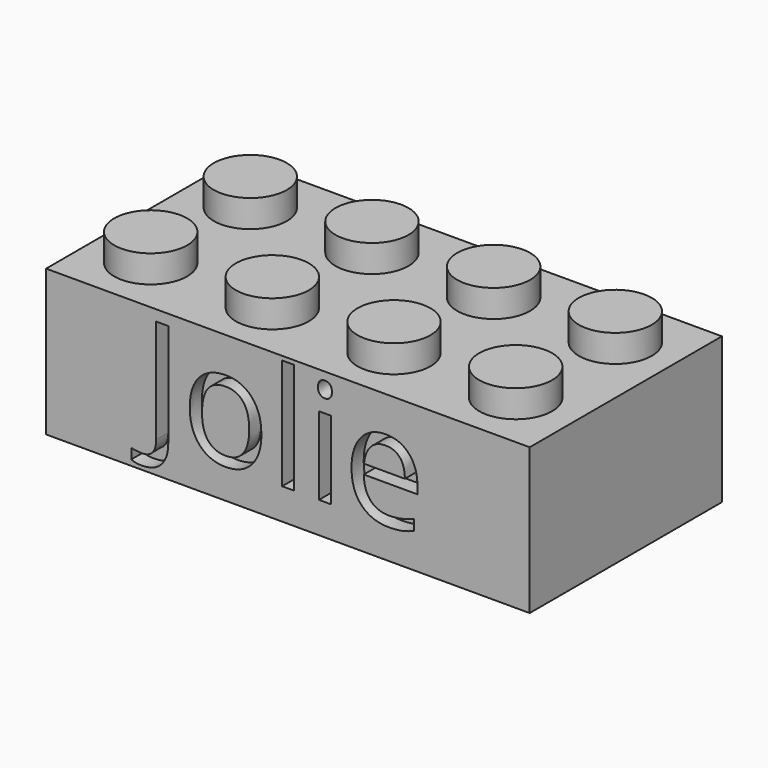
from build123d import *

# Parameters (mm, degrees)
F0_W          = 31.8
F0_H          = 15.8
F1_DEPTH      = 9.6
F2_W          = 29.4
F2_H          = 13.4
F3_DEPTH      = 8.4
F4_R          = 2.4
F5_DEPTH      = 1.8
F7_R          = 1.3
F8_DEPTH      = 1.2
F9_R          = 3.255
F9_R_2        = 2.4
F10_DEPTH     = 8.4
F11_W         = 0.6
F11_H         = 0.3
F12_DEPTH     = 9.6
F15_TEXT_SIZE = 9.5833333333
F16_DEPTH     = 1


# Not quite as in the source:
# - the program builds the solid bodies; features that only make, move or delete a surface that nothing else refers to are left out
# - Text() gives the source's letters only with a copy of the font that has no kerning and outlines rounded to 1/6400 em; it was checked with that copy


with BuildPart() as f1:
    # F0 (on Top) → F1 (new body)
    with BuildSketch(Plane.XY):
        Rectangle(F0_W, F0_H)
    extrude(amount=F1_DEPTH)

    # F2 (on Top) → F3 (cut)
    with BuildSketch(Plane.XY):
        Rectangle(F2_W, F2_H)
    extrude(amount=F3_DEPTH, mode=Mode.SUBTRACT)

    # F4 (on face) → F5 (join)
    with BuildSketch(Plane.XY.offset(9.6)):
        with Locations((-11.95, 3.95)):
            Circle(F4_R)
        with Locations((-12.1022495041, -4.0485511243)):
            Circle(F4_R)
        with Locations((-3.95, 3.95)):
            Circle(F4_R)
        with Locations((-4.1022495041, -4.0485511243)):
            Circle(F4_R)
        with Locations((4.05, 3.95)):
            Circle(F4_R)
        with Locations((3.8977504959, -4.0485511243)):
            Circle(F4_R)
        with Locations((12.05, 3.95)):
            Circle(F4_R)
        with Locations((11.8977504959, -4.0485511243)):
            Circle(F4_R)
    extrude(amount=F5_DEPTH)

    # F7 (on offset) → F8 (cut)
    with BuildSketch(Plane.XY.offset(8.4)):
        with Locations((-11.95, -3.95)):
            Circle(F7_R)
        with Locations((-11.95, 4.05)):
            Circle(F7_R)
        with Locations((-3.95, -3.95)):
            Circle(F7_R)
        with Locations((-3.95, 4.05)):
            Circle(F7_R)
        with Locations((4.05, -3.95)):
            Circle(F7_R)
        with Locations((4.05, 4.05)):
            Circle(F7_R)
        with Locations((12.05, -3.95)):
            Circle(F7_R)
        with Locations((12.05, 4.05)):
            Circle(F7_R)
    extrude(amount=F8_DEPTH, mode=Mode.SUBTRACT)

    # F11 (on face) → F12 (join)
    with BuildSketch(Plane.XY):
        with Locations((-11.95, -6.55)):
            Rectangle(F11_W, F11_H)
        with Locations((-3.95, -6.55)):
            Rectangle(F11_W, F11_H)
        with Locations((4.05, -6.55)):
            Rectangle(F11_W, F11_H)
        with Locations((12.05, -6.55)):
            Rectangle(F11_W, F11_H)
        with Locations((-11.9024184093, 6.55)):
            Rectangle(F11_W, F11_H)
        with Locations((-3.9024184093, 6.55)):
            Rectangle(F11_W, F11_H)
        with Locations((4.0975815907, 6.55)):
            Rectangle(F11_W, F11_H)
        with Locations((12.0975815907, 6.55)):
            Rectangle(F11_W, F11_H)
    extrude(amount=F12_DEPTH)

    # F15 (on face) → F16 (cut)
    with BuildSketch(Plane.XZ.offset(7.9)):
        with Locations((-9.5501027778, 2.0499226451)):
            Text('Jolie', F15_TEXT_SIZE, font='Open Sans', text_align=(TextAlign.LEFT, TextAlign.BOTTOM))
    extrude(amount=-F16_DEPTH, mode=Mode.SUBTRACT)


with BuildPart() as f10:
    # F9 (on offset) → F10 (new body, through all)
    with BuildSketch(Plane.XY.offset(8.4)):
        with Locations((-7.95, 0.05)):
            Circle(F9_R)
        with Locations((-7.95, 0.05)):
            Circle(F9_R_2, mode=Mode.SUBTRACT)
    extrude(amount=-F10_DEPTH)


with BuildPart() as f10b:
    # F9 (on offset) → F10, piece 2 (new body, through all)
    with BuildSketch(Plane.XY.offset(8.4)):
        with Locations((8.05, 0.05)):
            Circle(F9_R)
        with Locations((8.05, 0.05)):
            Circle(F9_R_2, mode=Mode.SUBTRACT)
    extrude(amount=-F10_DEPTH)


with BuildPart() as f10c:
    # F9 (on offset) → F10, piece 3 (new body, through all)
    with BuildSketch(Plane.XY.offset(8.4)):
        Circle(F9_R)
        Circle(F9_R_2, mode=Mode.SUBTRACT)
    extrude(amount=-F10_DEPTH)


solid = Compound([f1.part, f10.part, f10b.part, f10c.part])
